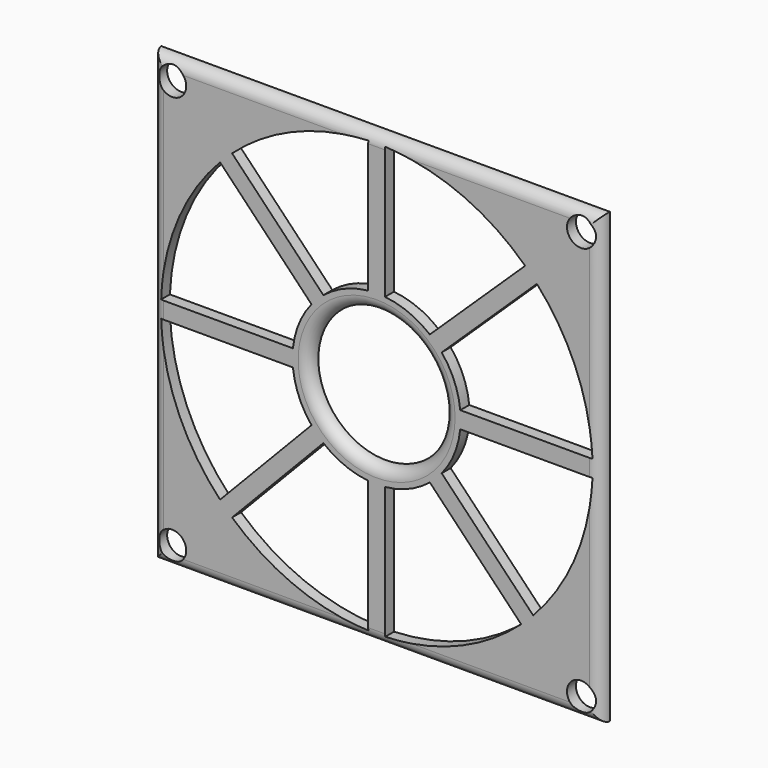
from build123d import *

# Parameters (mm, degrees)
F0_W        = 80
F0_H        = 80
F0_R        = 2.5
F0_R_2      = 12
F1_DEPTH    = 2
F2_T1_DEPTH = 90
F2_T3_DEPTH = 90


# Not quite as in the source:
# - a fillet or chamfer that OpenCascade refuses, or shapes differently, is made with other operations: its cross-section is extruded or revolved along the edge and cut away or added


with BuildPart() as f1:
    # F0 (on Front) → F1 (new body)
    with BuildSketch(Plane.XZ):
        with Locations((-0.0017476827, 0.1713572443)):
            Rectangle(F0_W, F0_H)
        with Locations((-36.4662137768, -36.2931088498)):
            Circle(F0_R, mode=Mode.SUBTRACT)
        with Locations((36.4627184114, -36.2931088498)):
            Circle(F0_R, mode=Mode.SUBTRACT)
        with Locations((-36.4662137768, 36.6358233383)):
            Circle(F0_R, mode=Mode.SUBTRACT)
        with BuildLine():
            ThreePointArc((38.4690204407, 1.6713572443), (38.4909436544, 0.9214996478), (38.4982523173, 0.1713572443))
            ThreePointArc((38.4982523173, 0.1713572443), (38.4909464293, -0.5786427557), (38.4690315381, -1.3283581108))
            ThreePointArc((38.4690315381, -1.3283581108), (35.4737380316, -14.7865808935), (27.9287857338, -26.3264785744))
            ThreePointArc((27.9287857338, -26.3264785744), (26.8753996766, -27.3943633128), (25.7812151161, -28.4204043195))
            ThreePointArc((25.7812151161, -28.4204043195), (14.5064210867, -35.4904295724), (1.498122464, -38.2994159419))
            ThreePointArc((1.498122464, -38.2994159419), (0.7484071972, -38.3213338497), (-0.0015927734, -38.3286427554))
            ThreePointArc((-0.0015927734, -38.3286427554), (-0.7517476827, -38.3213368677), (-1.5016178294, -38.2994159419))
            ThreePointArc((-1.5016178294, -38.2994159419), (-14.5093699729, -35.4906518899), (-25.7838341949, -28.421194497))
            ThreePointArc((-25.7838341949, -28.421194497), (-26.8780502008, -27.3951870251), (-27.9314689858, -26.3273345712))
            ThreePointArc((-27.9314689858, -26.3273345712), (-35.4773135858, -14.7863907098), (-38.4725889134, -1.3267665824))
            ThreePointArc((-38.4725889134, -1.3267665824), (-38.4944573001, -0.5778465387), (-38.5017476827, 0.1713572443))
            ThreePointArc((-38.5017476827, 0.1713572443), (-38.4944390198, 0.9214996478), (-38.472515806, 1.6713572443))
            ThreePointArc((-38.472515806, 1.6713572443), (-35.4771780599, 15.1294266234), (-27.9322810992, 26.6691930629))
            ThreePointArc((-27.9322810992, 26.6691930629), (-26.878895042, 27.7370778013), (-25.7847104814, 28.763118808))
            ThreePointArc((-25.7847104814, 28.763118808), (-14.5098447074, 35.8331732485), (-1.5014630377, 38.642136465))
            ThreePointArc((-1.5014630377, 38.642136465), (-0.7517476827, 38.6640513563), (-0.0017476827, 38.6713572443))
            ThreePointArc((-0.0017476827, 38.6713572443), (0.7482523173, 38.6640513563), (1.4979676723, 38.642136465))
            ThreePointArc((1.4979676723, 38.642136465), (14.9561904551, 35.6468429586), (26.4960881359, 28.1018906607))
            ThreePointArc((26.4960881359, 28.1018906607), (27.5639728743, 27.0485046035), (28.5900138811, 25.954320043))
            ThreePointArc((28.5900138811, 25.954320043), (35.6600146487, 14.6795861996), (38.4690204407, 1.6713572443))
        make_face(mode=Mode.SUBTRACT)
        with Locations((36.4627184114, 36.6358233383)):
            Circle(F0_R, mode=Mode.SUBTRACT)
        with BuildLine():
            Line((-9.495982875, 11.7842594703), (-25.7847104814, 28.763118808))
            ThreePointArc((-25.7847104814, 28.763118808), (-26.878895042, 27.7370778013), (-27.9322810992, 26.6691930629))
            Line((-27.9322810992, 26.6691930629), (-11.6157607218, 9.6642335801))
            ThreePointArc((-11.6157607218, 9.6642335801), (-10.608969906, 10.7773384203), (-9.495982875, 11.7842594703))
        make_face()
        with BuildLine():
            ThreePointArc((14.9230924791, -1.3283581108), (14.9794505742, -0.5794415216), (14.9982523173, 0.1713572443))
            ThreePointArc((14.9982523173, 0.1713572443), (14.979443414, 0.9222988702), (14.9230638739, 1.6713572443))
            ThreePointArc((14.9230638739, 1.6713572443), (13.8560844811, 5.9124797581), (11.6111545434, 9.6655924366))
            ThreePointArc((11.6111545434, 9.6655924366), (10.6042334933, 10.7785794675), (9.4911286531, 11.7853702834))
            ThreePointArc((9.4911286531, 11.7853702834), (5.7376930398, 14.0298860332), (1.496376144, 15.0963572443))
            ThreePointArc((1.496376144, 15.0963572443), (0.7482523173, 15.1525955108), (-0.0017476827, 15.1713572443))
            ThreePointArc((-0.0017476827, 15.1713572443), (-0.7517476827, 15.1525955108), (-1.4998715093, 15.0963572443))
            ThreePointArc((-1.4998715093, 15.0963572443), (-5.7419991682, 14.0295502319), (-9.495982875, 11.7842594703))
            ThreePointArc((-9.495982875, 11.7842594703), (-10.608969906, 10.7773384203), (-11.6157607218, 9.6642335801))
            ThreePointArc((-11.6157607218, 9.6642335801), (-13.8599156987, 5.9116690162), (-14.9265592393, 1.6713572443))
            ThreePointArc((-14.9265592393, 1.6713572443), (-14.9829387793, 0.9222988702), (-15.0017476827, 0.1713572443))
            ThreePointArc((-15.0017476827, 0.1713572443), (-14.9829859493, -0.5786427557), (-14.9267476827, -1.3267665824))
            ThreePointArc((-14.9267476827, -1.3267665824), (-13.8599406704, -5.5688942412), (-11.6146499088, -9.3228779481))
            ThreePointArc((-11.6146499088, -9.3228779481), (-10.6083494005, -10.4352444735), (-9.495982875, -11.4415449818))
            ThreePointArc((-9.495982875, -11.4415449818), (-5.7428099115, -13.6864998947), (-1.5016178294, -14.7534673625))
            ThreePointArc((-1.5016178294, -14.7534673625), (-0.7525467792, -14.8098409961), (-0.0015927734, -14.8286427549))
            ThreePointArc((-0.0015927734, -14.8286427549), (0.7492061289, -14.8098332416), (1.498122464, -14.7534673625))
            ThreePointArc((1.498122464, -14.7534673625), (5.7393145462, -13.6864998947), (9.4924875096, -11.4415449818))
            ThreePointArc((9.4924875096, -11.4415449818), (10.6054745406, -10.4346239318), (11.6122653564, -9.3215190916))
            ThreePointArc((11.6122653564, -9.3215190916), (13.8564750721, -5.5688223766), (14.9230924791, -1.3283581108))
        make_face()
        with Locations((-0.0017476827, 0.1713572443)):
            Circle(F0_R_2, mode=Mode.SUBTRACT)
        with BuildLine():
            Line((-0.0017476827, 15.1713572443), (-0.0017476827, 38.6713572443))
            ThreePointArc((-0.0017476827, 38.6713572443), (-0.7517476827, 38.6640513563), (-1.5014630377, 38.642136465))
            Line((-1.5014630377, 38.642136465), (-1.4998715093, 15.0963572443))
            ThreePointArc((-1.4998715093, 15.0963572443), (-0.7517476827, 15.1525955108), (-0.0017476827, 15.1713572443))
        make_face()
        with BuildLine():
            Line((1.496376144, 15.0963572443), (1.4979676723, 38.642136465))
            ThreePointArc((1.4979676723, 38.642136465), (0.7482523173, 38.6640513563), (-0.0017476827, 38.6713572443))
            Line((-0.0017476827, 38.6713572443), (-0.0017476827, 15.1713572443))
            ThreePointArc((-0.0017476827, 15.1713572443), (0.7482523173, 15.1525955108), (1.496376144, 15.0963572443))
        make_face()
        with BuildLine():
            Line((11.6111545434, 9.6655924366), (28.5900138811, 25.954320043))
            ThreePointArc((28.5900138811, 25.954320043), (27.5639728743, 27.0485046035), (26.4960881359, 28.1018906607))
            Line((26.4960881359, 28.1018906607), (9.4911286531, 11.7853702834))
            ThreePointArc((9.4911286531, 11.7853702834), (10.6042334933, 10.7785794675), (11.6111545434, 9.6655924366))
        make_face()
        with BuildLine():
            Line((14.9982523173, 0.1713572443), (38.4982523173, 0.1713572443))
            ThreePointArc((38.4982523173, 0.1713572443), (38.4909436544, 0.9214996478), (38.4690204407, 1.6713572443))
            Line((38.4690204407, 1.6713572443), (14.9230638739, 1.6713572443))
            ThreePointArc((14.9230638739, 1.6713572443), (14.979443414, 0.9222988702), (14.9982523173, 0.1713572443))
        make_face()
        with BuildLine():
            ThreePointArc((38.4690315381, -1.3283581108), (38.4909464293, -0.5786427557), (38.4982523173, 0.1713572443))
            Line((38.4982523173, 0.1713572443), (14.9982523173, 0.1713572443))
            ThreePointArc((14.9982523173, 0.1713572443), (14.9794505742, -0.5794415216), (14.9230924791, -1.3283581108))
            Line((14.9230924791, -1.3283581108), (38.4690315381, -1.3283581108))
        make_face()
        with BuildLine():
            ThreePointArc((25.7812151161, -28.4204043195), (26.8753996766, -27.3943633128), (27.9287857338, -26.3264785744))
            Line((27.9287857338, -26.3264785744), (11.6122653564, -9.3215190916))
            ThreePointArc((11.6122653564, -9.3215190916), (10.6054745406, -10.4346239318), (9.4924875096, -11.4415449818))
            Line((9.4924875096, -11.4415449818), (25.7812151161, -28.4204043195))
        make_face()
        with BuildLine():
            ThreePointArc((-0.0015927734, -38.3286427554), (0.7484071972, -38.3213338497), (1.498122464, -38.2994159419))
            Line((1.498122464, -38.2994159419), (1.498122464, -14.7534673625))
            ThreePointArc((1.498122464, -14.7534673625), (0.7492061289, -14.8098332416), (-0.0015927734, -14.8286427549))
            Line((-0.0015927734, -14.8286427549), (-0.0015927734, -38.3286427554))
        make_face()
        with BuildLine():
            ThreePointArc((-1.5016178294, -38.2994159419), (-0.7517476827, -38.3213368677), (-0.0015927734, -38.3286427554))
            Line((-0.0015927734, -38.3286427554), (-0.0015927734, -14.8286427549))
            ThreePointArc((-0.0015927734, -14.8286427549), (-0.7525467792, -14.8098409961), (-1.5016178294, -14.7534673625))
            Line((-1.5016178294, -14.7534673625), (-1.5016178294, -38.2994159419))
        make_face()
        with BuildLine():
            ThreePointArc((-27.9314689858, -26.3273345712), (-26.8780502008, -27.3951870251), (-25.7838341949, -28.421194497))
            Line((-25.7838341949, -28.421194497), (-9.495982875, -11.4415449818))
            ThreePointArc((-9.495982875, -11.4415449818), (-10.6083494005, -10.4352444735), (-11.6146499088, -9.3228779481))
            Line((-11.6146499088, -9.3228779481), (-27.9314689858, -26.3273345712))
        make_face()
        with BuildLine():
            ThreePointArc((-38.5017476827, 0.1713572443), (-38.4944573001, -0.5778465387), (-38.4725889134, -1.3267665824))
            Line((-38.4725889134, -1.3267665824), (-14.9267476827, -1.3267665824))
            ThreePointArc((-14.9267476827, -1.3267665824), (-14.9829859493, -0.5786427557), (-15.0017476827, 0.1713572443))
            Line((-15.0017476827, 0.1713572443), (-38.5017476827, 0.1713572443))
        make_face()
        with BuildLine():
            Line((-14.9265592393, 1.6713572443), (-38.472515806, 1.6713572443))
            ThreePointArc((-38.472515806, 1.6713572443), (-38.4944390198, 0.9214996478), (-38.5017476827, 0.1713572443))
            Line((-38.5017476827, 0.1713572443), (-15.0017476827, 0.1713572443))
            ThreePointArc((-15.0017476827, 0.1713572443), (-14.9829387793, 0.9222988702), (-14.9265592393, 1.6713572443))
        make_face()
    extrude(amount=F1_DEPTH)

    # F2: fillet of radius 2 on 5 edges, made by hand

    # F2_s2 → F2_t1 (cut)
    with BuildSketch(Plane.YZ.offset(-45.0017476827)):
        with BuildLine():
            ThreePointArc((0, 40.1713572443), (-1.4142135624, 39.5855708066), (-2, 38.1713572443))
            Line((-2, 38.1713572443), (-2, 40.1713572443))
            Line((-2, 40.1713572443), (0, 40.1713572443))
        make_face()
        with BuildLine():
            ThreePointArc((0, -39.8286427557), (-1.4142135624, -39.2428563181), (-2, -37.8286427557))
            Line((-2, -37.8286427557), (-2, -39.8286427557))
            Line((-2, -39.8286427557), (0, -39.8286427557))
        make_face()
    extrude(amount=F2_T1_DEPTH, mode=Mode.SUBTRACT)

    # F2_s4 → F2_t3 (cut)
    with BuildSketch(Plane.XY.offset(-44.8286427557)):
        with BuildLine():
            ThreePointArc((39.9982523173, 0), (39.4124658797, -1.4142135624), (37.9982523173, -2))
            Line((37.9982523173, -2), (39.9982523173, -2))
            Line((39.9982523173, -2), (39.9982523173, 0))
        make_face()
        with BuildLine():
            ThreePointArc((-40.0017476827, 0), (-39.4159612451, -1.4142135624), (-38.0017476827, -2))
            Line((-38.0017476827, -2), (-40.0017476827, -2))
            Line((-40.0017476827, -2), (-40.0017476827, 0))
        make_face()
    extrude(amount=F2_T3_DEPTH, mode=Mode.SUBTRACT)

    # F2_s5 → F2_t6 (revolve, cut)
    with BuildSketch(Plane.XY.offset(0.1713572443)):
        with BuildLine():
            ThreePointArc((11.9982523173, 0), (12.5840387549, -1.4142135624), (13.9982523173, -2))
            Line((13.9982523173, -2), (11.9982523173, -2))
            Line((11.9982523173, -2), (11.9982523173, 0))
        make_face()
    revolve(axis=Axis((-0.0017476827, -2, 0.1713572443), (0, -1, 0)), mode=Mode.SUBTRACT)


solid = f1.part
